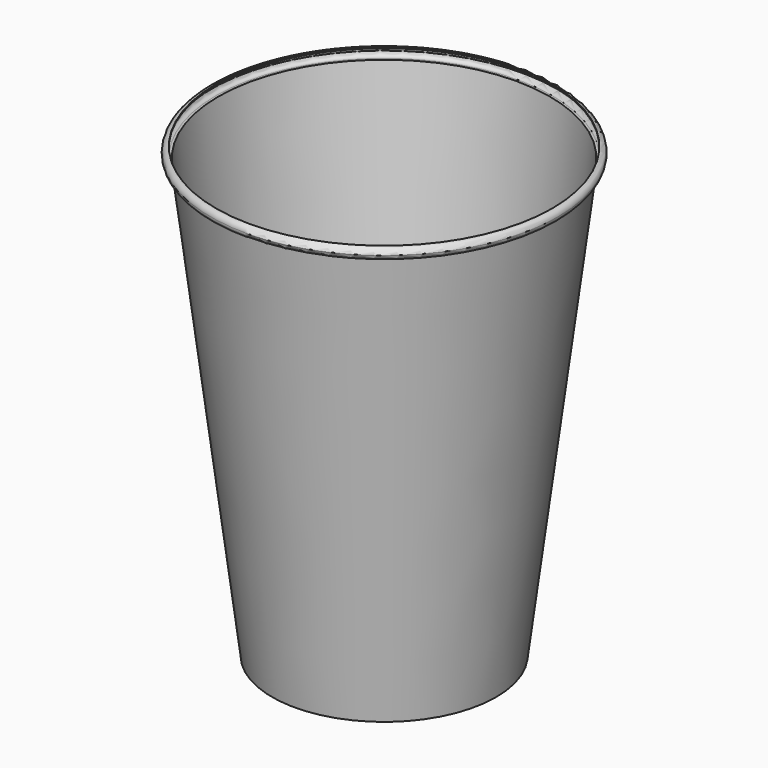
from build123d import *

# Parameters (mm, degrees)
F2_R     = 25.4
F0_R     = 38.1
F3_R     = 24.13
F5_DEPTH = 3.175
F6_R     = 39.37
F7_DEPTH = 2.54
F8_R     = 1.26999
F9_T     = -0.254


# Not quite as in the source:
# - a fillet or chamfer is up to 0.001 mm smaller than in the source, because OpenCascade refuses the exact size
# - a shell that OpenCascade refuses in one call is made with other operations: the cavity is built on its own and cut out


with BuildPart() as f4:
    # F2 (on offset) → F4 section 0
    with BuildSketch(Plane.XY.offset(-101.6)):
        Circle(F2_R)
    # F0 (on Top) → F4 section 1
    with BuildSketch(Plane.XY):
        Circle(F0_R)
    loft()

    # F3 (on offset) → F5 (cut)
    with BuildSketch(Plane.XY.offset(-101.6)):
        Circle(F3_R)
    extrude(amount=F5_DEPTH, mode=Mode.SUBTRACT)

    # F6 (on Top) → F7 (join)
    with BuildSketch(Plane.XY):
        Circle(F6_R)
    extrude(amount=-F7_DEPTH)

    # F8 (radius 1.27 in the source; OpenCascade refuses exactly that, so slightly less here)
    f8_edges = [f4.edges().sort_by_distance(p)[0] for p in [
        (-39.37, 0, -2.54),
        (-39.37, 0, 0),
    ]]
    fillet(f8_edges, radius=F8_R)

    # F9: a shell. OpenCascade refuses it in one call, so the cavity is built on its own and cut out:
    # the body offset inwards by the wall thickness, plus a prism from it out through each open face.
    f9_core = offset(f4.part, amount=F9_T, kind=Kind.INTERSECTION, mode=Mode.PRIVATE)
    f9_exits = [f9_core.faces().sort_by_distance(p)[0] for p in [
        (0, 0, -0.254),
    ]]
    add(f9_core, mode=Mode.SUBTRACT)
    extrude(f9_exits, amount=-F9_T, mode=Mode.SUBTRACT)


solid = f4.part
